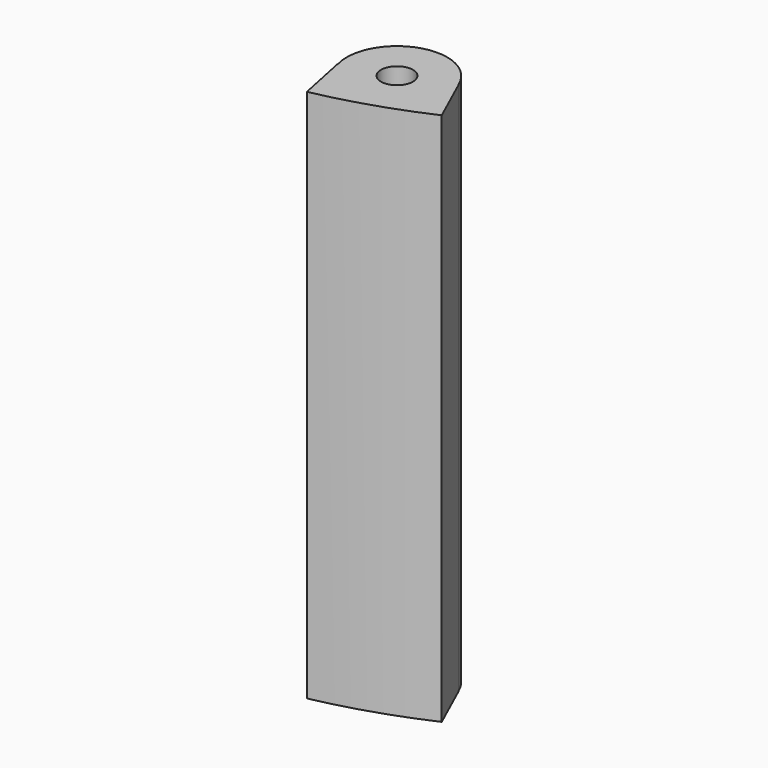
from build123d import *

# Parameters (mm, degrees)
F0_R     = 1.5
F1_DEPTH = 50


# Not quite as in the source:
# - ends of sketch curves that miss each other by under 0.0002 mm in the source are joined


with BuildPart() as f1:
    # F0 (on Top) → F1 (new body)
    with BuildSketch(Plane.XY):
        with BuildLine():
            Line((-5.449118, -0.504862), (-4.441162, -5.402211))
            ThreePointArc((-4.441162, -5.402211), (0.6615584195, -4.0525834634), (5.5830371113, -2.1451512457))
            Line((5.5830371113, -2.1451512457), (3.519902, 2.409349))
            Line((3.519902, 2.409349), (3.498846, 2.399818))
            ThreePointArc((3.498846, 2.399818), (0.6786519051, 5.1349674747), (-3.2332818366, 4.772594717))
            ThreePointArc((-3.2332818366, 4.772594717), (-5.2226446667, 2.5075404986), (-5.4264814855, -0.5001971285))
            Line((-5.4264814855, -0.5001971285), (-5.449118, -0.504862))
        make_face()
        with Locations((-0.883526, 0.702699)):
            Circle(F0_R, mode=Mode.SUBTRACT)
    extrude(amount=F1_DEPTH)


solid = f1.part
